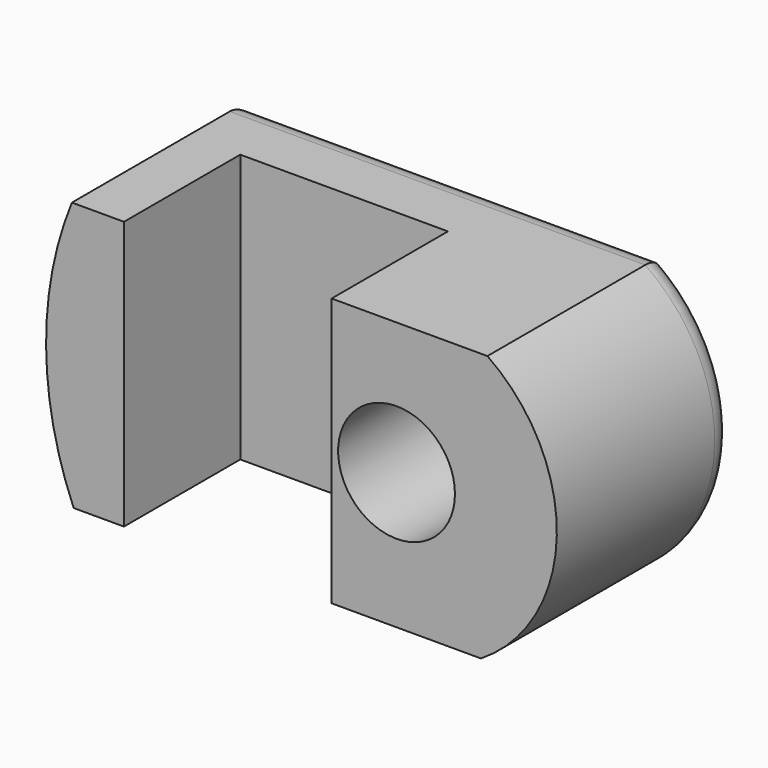
from build123d import *

# Parameters (mm, degrees)
F1_DEPTH    = 5.6
F0_R        = 2.25
F0_W        = 8
F0_H        = 10.336498642
F2_DEPTH    = 3
F3_T1_DEPTH = 20.6876119668
F3_T3_DEPTH = 21.0057116197
F3_T6_ANGLE = 66.24239892
F3_T8_ANGLE = 176.3763770041


# Not quite as in the source:
# - a fillet or chamfer that OpenCascade refuses, or shapes differently, is made with other operations: its cross-section is extruded or revolved along the edge and cut away or added


with BuildPart() as f1:
    # F0 (on Front) → F1 (new body)
    with BuildSketch(Plane.XZ):
        with BuildLine():
            Line((-10.5, 5.086498642), (-12.5051002221, 5.086498642))
            ThreePointArc((-12.5051002221, 5.086498642), (-13.4997099623, -0.0884925705), (-12.4373429638, -5.25))
            Line((-12.4373429638, -5.25), (-10.5, -5.25))
            Line((-10.5, -5.25), (-10.5, 5.086498642))
        make_face()
    extrude(amount=F1_DEPTH)



with BuildPart() as f1b:
    # F0 (on Front) → F1, piece 2 (new body)
    with BuildSketch(Plane.XZ):
        with BuildLine():
            Line((3.5006113976, 5.086498642), (-2.5, 5.086498642))
            Line((-2.5, 5.086498642), (-2.5, -5.25))
            Line((-2.5, -5.25), (3.2502690029, -5.25))
            ThreePointArc((3.2502690029, -5.25), (6.1728759577, -0.1495025156), (3.5006113976, 5.086498642))
        make_face()
        Circle(F0_R, mode=Mode.SUBTRACT)
    extrude(amount=F1_DEPTH)


with BuildPart() as f1_1:
    add(f1.part)

    add(f1b.part)  # F2 merges F1b
    # F0 (on Front) → F2 (join)
    with BuildSketch(Plane.XZ):
        with BuildLine():
            Line((-10.5, 5.086498642), (-12.5051002221, 5.086498642))
            ThreePointArc((-12.5051002221, 5.086498642), (-13.4997099623, -0.0884925705), (-12.4373429638, -5.25))
            Line((-12.4373429638, -5.25), (-10.5, -5.25))
            Line((-10.5, -5.25), (-10.5, 5.086498642))
        make_face()
        with Locations((-6.5, -0.081750679)):
            Rectangle(F0_W, F0_H)
        with BuildLine():
            Line((3.5006113976, 5.086498642), (-2.5, 5.086498642))
            Line((-2.5, 5.086498642), (-2.5, -5.25))
            Line((-2.5, -5.25), (3.2502690029, -5.25))
            ThreePointArc((3.2502690029, -5.25), (6.1728759577, -0.1495025156), (3.5006113976, 5.086498642))
        make_face()
        Circle(F0_R, mode=Mode.SUBTRACT)
    extrude(amount=-F2_DEPTH)

    # F3: fillet of radius 1 on 4 edges, made by hand

    # F3_s2 → F3_t1 (cut)
    with BuildSketch(Plane.YZ.offset(-14.9373429638)):
        with BuildLine():
            ThreePointArc((3, -4.25), (2.7071067812, -4.9571067812), (2, -5.25))
            Line((2, -5.25), (3, -5.25))
            Line((3, -5.25), (3, -4.25))
        make_face()
    extrude(amount=F3_T1_DEPTH, mode=Mode.SUBTRACT)

    # F3_s4 → F3_t3 (cut)
    with BuildSketch(Plane.YZ.offset(-15.0051002221)):
        with BuildLine():
            ThreePointArc((3, 4.086498642), (2.7071067812, 4.7936054231), (2, 5.086498642))
            Line((2, 5.086498642), (3, 5.086498642))
            Line((3, 5.086498642), (3, 4.086498642))
        make_face()
    extrude(amount=F3_T3_DEPTH, mode=Mode.SUBTRACT)

    # F3_s5 → F3_t6 (revolve, cut)
    with BuildSketch(Plane(origin=(0, 0, 0), x_dir=(0, 1, 0), z_dir=(0.5409102149, 0, 0.8410803406))):
        with BuildLine():
            ThreePointArc((3, 12.5), (2.7071067812, 13.2071067812), (2, 13.5))
            Line((2, 13.5), (3, 13.5))
            Line((3, 13.5), (3, 12.5))
        make_face()
    revolve(axis=Axis((0, 3, 0), (0, -1, 0)), revolution_arc=F3_T6_ANGLE, mode=Mode.SUBTRACT)

    # F3_s7 → F3_t8 (revolve, cut)
    with BuildSketch(Plane(origin=(0, 0, 0), x_dir=(0, 1, 0), z_dir=(-0.9888894164, 0, -0.148653026))):
        with BuildLine():
            ThreePointArc((2, 6.1746861128), (2.7071067812, 5.881792894), (3, 5.1746861128))
            Line((3, 5.1746861128), (3, 6.1746861128))
            Line((3, 6.1746861128), (2, 6.1746861128))
        make_face()
    revolve(axis=Axis((0, 3, 0), (0, -1, 0)), revolution_arc=F3_T8_ANGLE, mode=Mode.SUBTRACT)


solid = f1_1.part
